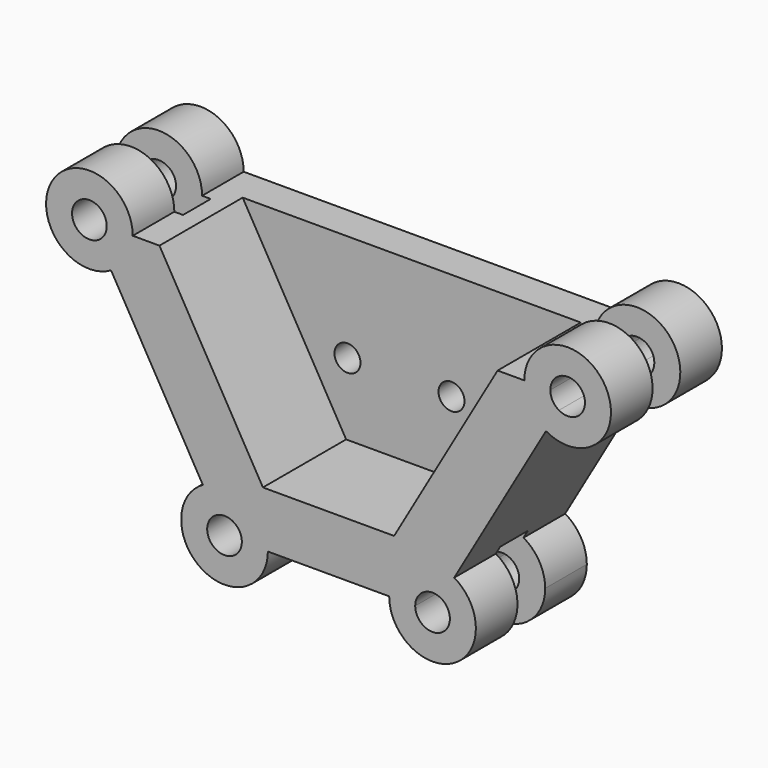
from build123d import *

# Parameters (mm, degrees)
F1_DEPTH = 50.8
F3_DEPTH = 76.2
F4_R     = 38.1
F5_DEPTH = 12.7
F6_R     = 9.525
F7_DEPTH = 25.401


with BuildPart() as f1:
    # F0 (on Front) → F1 (new body, symmetric)
    with BuildSketch(Plane.XZ):
        with BuildLine():
            ThreePointArc((-83.1071616711, -65.430798607), (-83.1071616711, -120.4234117473), (-35.4821616711, -92.9271051772))
            Line((-35.4821616711, -92.9271051772), (-54.5321616711, -92.9271051772))
            ThreePointArc((-54.5321616711, -92.9271051772), (-73.5821616711, -103.9256278052), (-73.5821616711, -81.9285825491))
            Line((-73.5821616711, -81.9285825491), (-83.1071616711, -65.430798607))
        make_face()
        with BuildLine():
            ThreePointArc((-83.1071616711, -65.430798607), (-51.3571616711, -65.430798607), (-35.4821616711, -92.9271051772))
            Line((-35.4821616711, -92.9271051772), (53.4178383289, -92.9271051772))
            ThreePointArc((53.4178383289, -92.9271051772), (69.2928383289, -65.430798607), (101.0428383289, -65.430798607))
            Line((101.0428383289, -65.430798607), (168.2795419814, 51.0265882527))
            ThreePointArc((168.2795419814, 51.0265882527), (156.6582354113, 62.6478948228), (152.4045419814, 78.5228948228))
            Line((152.4045419814, 78.5228948228), (-134.4688653237, 78.5228948228))
            ThreePointArc((-134.4688653237, 78.5228948228), (-138.7225587535, 62.6478948228), (-150.3438653237, 51.0265882527))
            Line((-150.3438653237, 51.0265882527), (-83.1071616711, -65.430798607))
        make_face()
        with BuildLine():
            Line((-54.5321616711, -92.9271051772), (-35.4821616711, -92.9271051772))
            ThreePointArc((-35.4821616711, -92.9271051772), (-51.3571616711, -65.430798607), (-83.1071616711, -65.430798607))
            Line((-83.1071616711, -65.430798607), (-73.5821616711, -81.9285825491))
            ThreePointArc((-73.5821616711, -81.9285825491), (-60.8821616711, -81.9285825491), (-54.5321616711, -92.9271051772))
        make_face()
        with BuildLine():
            ThreePointArc((101.0428383289, -65.430798607), (69.2928383289, -65.430798607), (53.4178383289, -92.9271051772))
            Line((53.4178383289, -92.9271051772), (72.4678383289, -92.9271051772))
            ThreePointArc((72.4678383289, -92.9271051772), (78.8178383289, -81.9285825491), (91.5178383289, -81.9285825491))
            Line((91.5178383289, -81.9285825491), (101.0428383289, -65.430798607))
        make_face()
        with BuildLine():
            Line((72.4678383289, -92.9271051772), (53.4178383289, -92.9271051772))
            ThreePointArc((53.4178383289, -92.9271051772), (85.1678383289, -124.6771051772), (116.9178383289, -92.9271051772))
            ThreePointArc((116.9178383289, -92.9271051772), (112.664144899, -77.0521051772), (101.0428383289, -65.430798607))
            Line((101.0428383289, -65.430798607), (91.5178383289, -81.9285825491))
            ThreePointArc((91.5178383289, -81.9285825491), (96.1663609569, -86.5771051772), (97.8678383289, -92.9271051772))
            ThreePointArc((97.8678383289, -92.9271051772), (85.1678383289, -105.6271051772), (72.4678383289, -92.9271051772))
        make_face()
        with BuildLine():
            ThreePointArc((-134.4688653237, 78.5228948228), (-193.7151718938, 94.3978948228), (-150.3438653237, 51.0265882527))
            Line((-150.3438653237, 51.0265882527), (-159.8688653237, 67.5243721948))
            ThreePointArc((-159.8688653237, 67.5243721948), (-177.2173879518, 84.8728948228), (-153.5188653237, 78.5228948228))
            Line((-153.5188653237, 78.5228948228), (-134.4688653237, 78.5228948228))
        make_face()
        with BuildLine():
            Line((-159.8688653237, 67.5243721948), (-150.3438653237, 51.0265882527))
            ThreePointArc((-150.3438653237, 51.0265882527), (-138.7225587535, 62.6478948228), (-134.4688653237, 78.5228948228))
            Line((-134.4688653237, 78.5228948228), (-153.5188653237, 78.5228948228))
            ThreePointArc((-153.5188653237, 78.5228948228), (-155.2203426956, 72.1728948228), (-159.8688653237, 67.5243721948))
        make_face()
        with BuildLine():
            ThreePointArc((152.4045419814, 78.5228948228), (156.6582354113, 62.6478948228), (168.2795419814, 51.0265882527))
            Line((168.2795419814, 51.0265882527), (177.8045419814, 67.5243721948))
            ThreePointArc((177.8045419814, 67.5243721948), (173.1560193534, 72.1728948228), (171.4545419814, 78.5228948228))
            Line((171.4545419814, 78.5228948228), (152.4045419814, 78.5228948228))
        make_face()
        with BuildLine():
            Line((177.8045419814, 67.5243721948), (168.2795419814, 51.0265882527))
            ThreePointArc((168.2795419814, 51.0265882527), (200.0295419814, 51.0265882527), (215.9045419814, 78.5228948228))
            ThreePointArc((215.9045419814, 78.5228948228), (184.1545419814, 110.2728948228), (152.4045419814, 78.5228948228))
            Line((152.4045419814, 78.5228948228), (171.4545419814, 78.5228948228))
            ThreePointArc((171.4545419814, 78.5228948228), (184.1545419814, 91.2228948228), (196.8545419814, 78.5228948228))
            ThreePointArc((196.8545419814, 78.5228948228), (190.5045419814, 67.5243721948), (177.8045419814, 67.5243721948))
        make_face()
    extrude(amount=F1_DEPTH, both=True)

    # F2 (on face) → F3 (cut)
    with BuildSketch(Plane.XZ.offset(50.8)):
        Polygon((132.8281030505, 78.5228948228), (-114.8924263927, 78.5228948228), (-39.0819515524, -52.7846993466), (57.0176282101, -52.7846993466), align=None)
    extrude(amount=-F3_DEPTH, mode=Mode.SUBTRACT)

    # F4 (on Front) → F5 (cut, symmetric)
    with BuildSketch(Plane.XZ):
        with Locations((-166.2188653237, 78.5228948228)):
            Circle(F4_R)
        with Locations((-67.2321616711, -92.9271051772)):
            Circle(F4_R)
        with Locations((85.1678383289, -92.9271051772)):
            Circle(F4_R)
        with Locations((184.1545419814, 78.5228948228)):
            Circle(F4_R)
    extrude(amount=F5_DEPTH, both=True, mode=Mode.SUBTRACT)

    # F6 (on face) → F7 (cut, through all)
    with BuildSketch(Plane.XZ.offset(-25.4)):
        with Locations((-38.1, 0)):
            Circle(F6_R)
        with Locations((38.1, 0)):
            Circle(F6_R)
    extrude(amount=-F7_DEPTH, mode=Mode.SUBTRACT)


solid = f1.part
